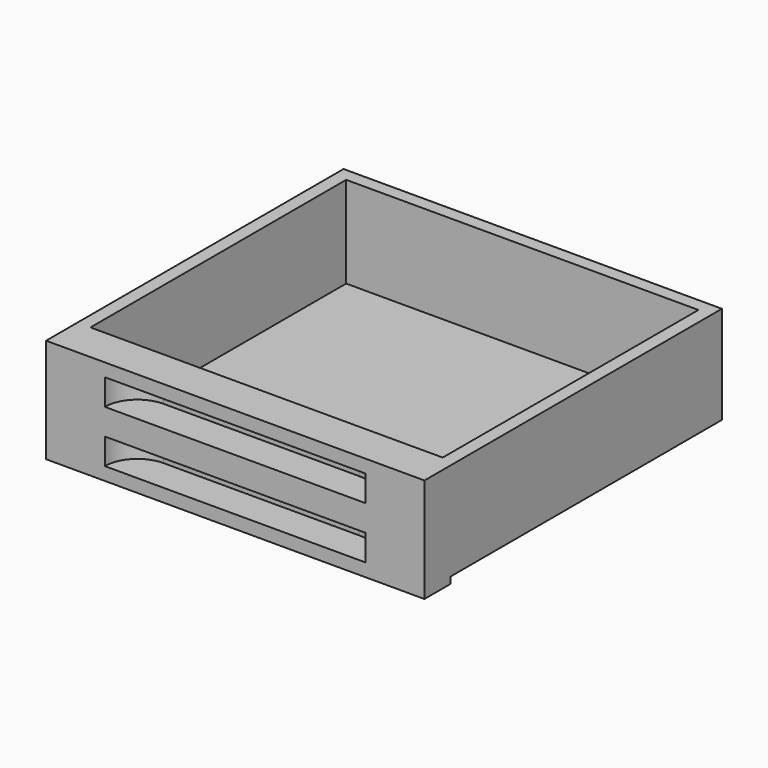
from build123d import *

# Parameters (mm, degrees)
F1_DEPTH = 57
F0_W     = 54
F0_H     = 14
F2_DEPTH = 2
F3_START = 51
F3_DEPTH = 6
F4_W     = 40
F4_H     = 4
F5_DEPTH = 5
F6_R     = 4.99999
F7_W     = 52
F7_H     = 1
F8_DEPTH = 2
F9_START = -56
F9_DEPTH = 2


# Not quite as in the source:
# - a fillet or chamfer is up to 0.001 mm smaller than in the source, because OpenCascade refuses the exact size


with BuildPart() as f1:
    # F0 (on Front) → F1 (new body)
    with BuildSketch(Plane.XZ):
        Polygon((-59.5397581918, 21.3998371276), (-61.5397581918, 21.3998371276), (-61.5397581918, 5.3998371276), (-3.5397581918, 5.3998371276), (-3.5397581918, 21.3998371276), (-5.5397581918, 21.3998371276), (-5.5397581918, 7.3998371276), (-59.5397581918, 7.3998371276), align=None)
    extrude(amount=F1_DEPTH)

    # F0 (on Front) → F2 (join)
    with BuildSketch(Plane.XZ):
        with Locations((-32.5397581918, 14.3998371276)):
            Rectangle(F0_W, F0_H)
    extrude(amount=F2_DEPTH)

    # F0 (on Front) → F3 (join)
    with BuildSketch(Plane.XZ.offset(F3_START)):
        with Locations((-32.5397581918, 14.3998371276)):
            Rectangle(F0_W, F0_H)
    extrude(amount=F3_DEPTH)

    # F4 (on face) → F5 (cut)
    with BuildSketch(Plane.XZ.offset(57)):
        with Locations((-32.5397581918, 17.3998371276)):
            Rectangle(F4_W, F4_H)
        with Locations((-32.5397581918, 9.3998371276)):
            Rectangle(F4_W, F4_H)
    extrude(amount=-F5_DEPTH, mode=Mode.SUBTRACT)

    # F6 (radius 5 in the source; OpenCascade refuses exactly that, so slightly less here)
    f6_edges = [f1.edges().sort_by_distance(p)[0] for p in [
        (-52.539758, -52, 17.399837),
        (-52.539758, -52, 9.399837),
        (-12.539758, -52, 17.399837),
        (-12.539758, -52, 9.399837),
    ]]
    fillet(f6_edges, radius=F6_R)

    # F7 (on face) → F8 (cut)
    with BuildSketch(Plane(origin=(-61.5397581918, 0, 0), x_dir=(0, -1, 0), z_dir=(-1, 0, 0))):
        with Locations((26, 5.8998371276)):
            Rectangle(F7_W, F7_H)
    extrude(amount=-F8_DEPTH, mode=Mode.SUBTRACT)

    # F7 (on face) → F9 (cut)
    with BuildSketch(Plane(origin=(-61.5397581918, 0, 0), x_dir=(0, -1, 0), z_dir=(-1, 0, 0)).offset(F9_START)):
        with Locations((26, 5.8998371276)):
            Rectangle(F7_W, F7_H)
    extrude(amount=-F9_DEPTH, mode=Mode.SUBTRACT)


solid = f1.part
